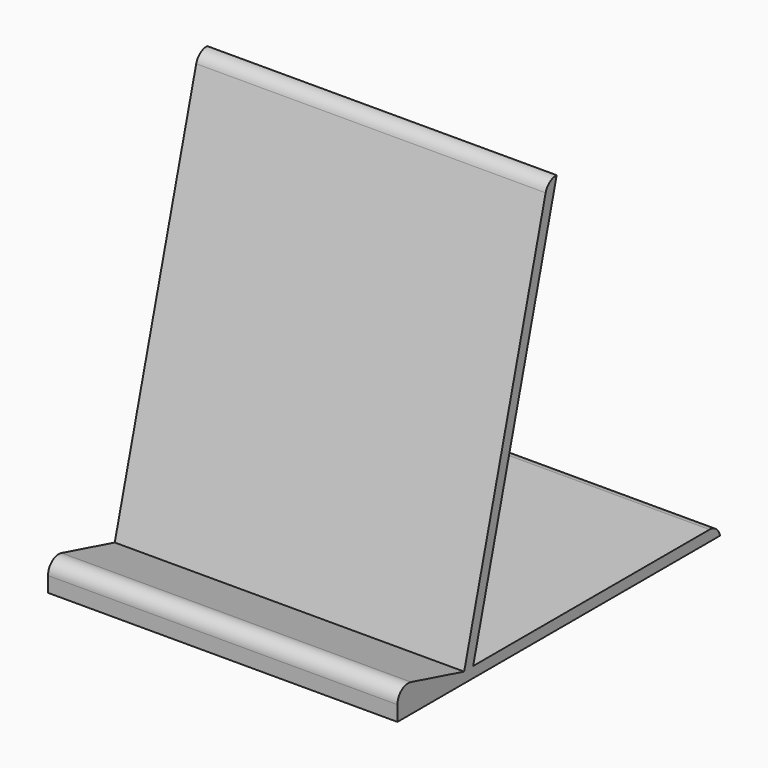
from build123d import *

# Parameters (mm, degrees)
F1_DEPTH    = 130
F2_T1_DEPTH = 154.4948974279
F3_T1_DEPTH = 154.4948974279
F4_R        = 5


# Not quite as in the source:
# - a fillet or chamfer that OpenCascade refuses, or shapes differently, is made with other operations: its cross-section is extruded or revolved along the edge and cut away or added


with BuildPart() as f1:
    # F0 (on Right) → F1 (new body)
    with BuildSketch(Plane.YZ):
        Polygon((1.0352761804, 3.8637033052), (0, 0), (120, 0), (120, 4), (5.2129014914, 4), (44.0560821698, 148.9647238196), (40.1923788647, 150), align=None)
        Polygon((-30, 0), (0, 0), (1.0352761804, 3.8637033052), (-30, 12.1795804946), (-30, 4.0079755444), align=None)
    extrude(amount=F1_DEPTH)

    # F2: fillet of radius 5 on 1 edges, made by hand

    # F2_s2 → F2_t1 (cut)
    with BuildSketch(Plane.YZ.offset(-12.2474487139)):
        with BuildLine():
            ThreePointArc((44.0560821698, 148.9647238196), (40.8315018491, 148.0307814801), (38.9244296722, 145.2679491924))
            Line((38.9244296722, 145.2679491924), (40.1923788647, 150))
            Line((40.1923788647, 150), (44.0560821698, 148.9647238196))
        make_face()
    extrude(amount=F2_T1_DEPTH, mode=Mode.SUBTRACT)

    # F3: fillet of radius 5 on 1 edges, made by hand

    # F3_s2 → F3_t1 (cut)
    with BuildSketch(Plane.YZ.offset(-12.2474487139)):
        with BuildLine():
            ThreePointArc((115.1010205144, 4), (118.2632981746, 2.8729833462), (120, 0))
            Line((120, 0), (120, 4))
            Line((120, 4), (115.1010205144, 4))
        make_face()
    extrude(amount=F3_T1_DEPTH, mode=Mode.SUBTRACT)

    # F4
    f4_edges = [f1.edges().sort_by_distance(p)[0] for p in [
        (65, -30, 12.17958),
    ]]
    fillet(f4_edges, radius=F4_R)


solid = f1.part
